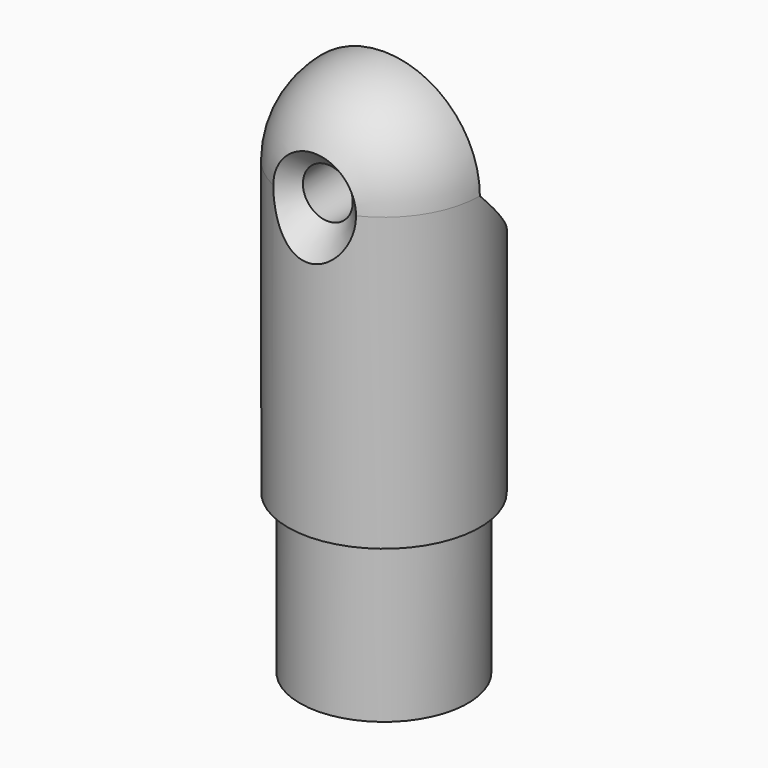
from build123d import *

# Parameters (mm, degrees)
F2_R           = 12.7
F3_DEPTH       = 12.701
F6_D           = 6.6
F6_CSINK_D     = 13.44
F6_CSINK_ANGLE = 90


# Not quite as in the source:
# - a length typed as a fraction of an inch, garbled in the dataset ("3 / 203.2 mm" for 3/8 in), is restored


with BuildPart() as f1:
    # F0 (on Front) → F1 (revolve)
    with BuildSketch(Plane.XZ):
        with BuildLine():
            Line((0, -46.4494958016), (0, 25.8821103648))
            ThreePointArc((0, 25.8821103648), (-8.9802561211, 22.1623664858), (-12.7, 13.1821103648))
            Line((-12.7, 13.1821103648), (-12.7, -25.4462463191))
            Line((-12.7, -25.4462463191), (-11.1125, -25.4462463191))
            Line((-11.1125, -25.4462463191), (-11.1125, -46.4494958016))
            Line((-11.1125, -46.4494958016), (0, -46.4494958016))
        make_face()
    revolve(axis=Axis((0, 0, -7.9082977027), (0, 0, -1)))

    # F2 (on Front) → F3 (cut, through all)
    with BuildSketch(Plane.XZ):
        with Locations((0, 13.1821103648)):
            Circle(F2_R)
    extrude(amount=-F3_DEPTH, mode=Mode.SUBTRACT)

    # F6 (through all)
    with Locations(Plane.XZ.offset(12.7)):
        with Locations((0, 13.1821103648)):
            CounterSinkHole(F6_D / 2, F6_CSINK_D / 2, counter_sink_angle=F6_CSINK_ANGLE)


solid = f1.part
